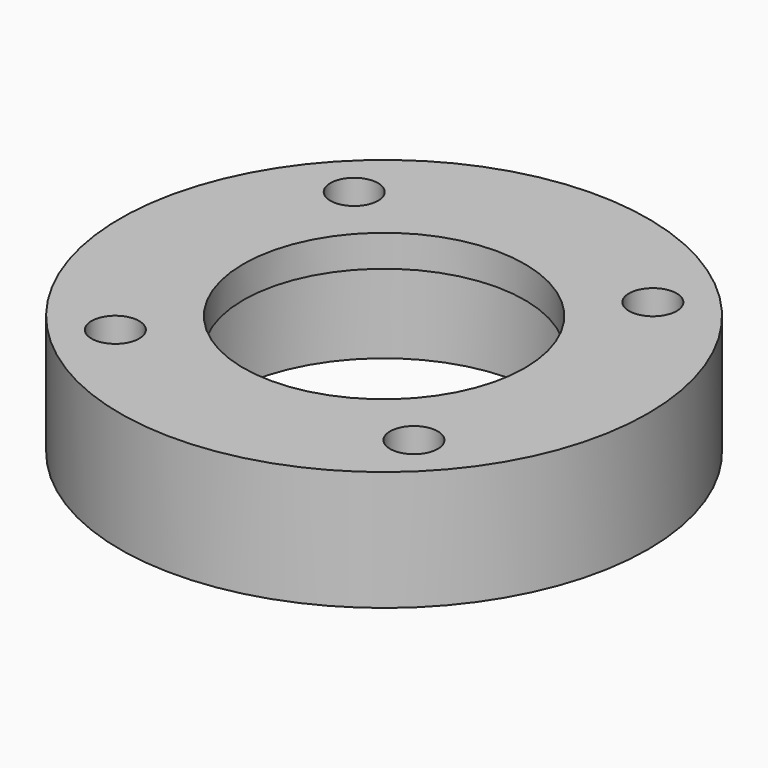
from build123d import *

# Parameters (mm, degrees)
F0_R            = 23.8125
F0_R_2          = 2.15265
F0_R_3          = 14.2875
F1_DEPTH        = 7.9375
F3_DEPTH        = 7.9375
F3_COPIES_COUNT = 4
F4_R            = 23.8125
F4_R_2          = 2.15265
F4_R_3          = 14.2875
F4_R_4          = 12.7
F5_DEPTH        = 2.8575


# Not quite as in the source:
# - a pattern or mirror of a feature is missing from the dataset's text; its kind, count and spacing are read off the source's solid


with BuildPart() as f1:
    # F0 (on Top) → F1 (new body)
    with BuildSketch(Plane.XY):
        Circle(F0_R)
        with Locations((-13.4703841816, -13.4703841816)):
            Circle(F0_R_2, mode=Mode.SUBTRACT)
        with Locations((13.4703841816, -13.4703841816)):
            Circle(F0_R_2, mode=Mode.SUBTRACT)
        with Locations((-13.4703841816, 13.4703841816)):
            Circle(F0_R_2, mode=Mode.SUBTRACT)
        Circle(F0_R_3, mode=Mode.SUBTRACT)
        with Locations((13.4703841816, 13.4703841816)):
            Circle(F0_R_2, mode=Mode.SUBTRACT)
    extrude(amount=F1_DEPTH)

    # F2 (on face) → F3 (cut, through all)
    with BuildSketch(Plane.XY.offset(7.9375)):
        with BuildLine():
            ThreePointArc((12.7805200237, -18.1826547271), (10.4181406182, -17.1262309344), (8.9569606825, -14.9903889737))
            ThreePointArc((8.9569606825, -14.9903889737), (0, -17.4625), (-8.9569606825, -14.9903889737))
            ThreePointArc((-8.9569606825, -14.9903889737), (-10.4181406182, -17.1262309344), (-12.7805200237, -18.1826547271))
            ThreePointArc((-12.7805200237, -18.1826547271), (0, -22.225), (12.7805200237, -18.1826547271))
        make_face()
    f3 = extrude(amount=-F3_DEPTH, mode=Mode.SUBTRACT)

    # F3_copies: F3 ×4 about axis
    f3_copies_axis = Axis((0, 0, 0), (0, 0, 1))
    for i in range(1, F3_COPIES_COUNT):
        add(f3.rotate(f3_copies_axis, i * 360 / F3_COPIES_COUNT), mode=Mode.SUBTRACT)

    # F4 (on face) → F5 (join)
    with BuildSketch(Plane.XY.offset(7.9375)):
        Circle(F4_R)
        with Locations((-13.4703841816, -13.4703841816)):
            Circle(F4_R_2, mode=Mode.SUBTRACT)
        with BuildLine():
            ThreePointArc((-8.9569606825, -14.9903889737), (0, -17.4625), (8.9569606825, -14.9903889737))
            ThreePointArc((8.9569606825, -14.9903889737), (10.4181406182, -17.1262309344), (12.7805200237, -18.1826547271))
            ThreePointArc((12.7805200237, -18.1826547271), (0, -22.225), (-12.7805200237, -18.1826547271))
            ThreePointArc((-12.7805200237, -18.1826547271), (-10.4181406182, -17.1262309344), (-8.9569606825, -14.9903889737))
        make_face(mode=Mode.SUBTRACT)
        with Locations((13.4703841816, -13.4703841816)):
            Circle(F4_R_2, mode=Mode.SUBTRACT)
        with BuildLine():
            ThreePointArc((-14.9903889737, 8.9569606825), (-17.4625, 0), (-14.9903889737, -8.9569606825))
            ThreePointArc((-14.9903889737, -8.9569606825), (-17.1262309344, -10.4181406182), (-18.1826547271, -12.7805200237))
            ThreePointArc((-18.1826547271, -12.7805200237), (-22.225, 0), (-18.1826547271, 12.7805200237))
            ThreePointArc((-18.1826547271, 12.7805200237), (-17.1262309344, 10.4181406182), (-14.9903889737, 8.9569606825))
        make_face(mode=Mode.SUBTRACT)
        with Locations((-13.4703841816, 13.4703841816)):
            Circle(F4_R_2, mode=Mode.SUBTRACT)
        Circle(F4_R_3, mode=Mode.SUBTRACT)
        with BuildLine():
            ThreePointArc((14.9903889737, -8.9569606825), (17.4625, 0), (14.9903889737, 8.9569606825))
            ThreePointArc((14.9903889737, 8.9569606825), (17.1262309344, 10.4181406182), (18.1826547271, 12.7805200237))
            ThreePointArc((18.1826547271, 12.7805200237), (22.225, 0), (18.1826547271, -12.7805200237))
            ThreePointArc((18.1826547271, -12.7805200237), (17.1262309344, -10.4181406182), (14.9903889737, -8.9569606825))
        make_face(mode=Mode.SUBTRACT)
        with BuildLine():
            ThreePointArc((8.9569606825, 14.9903889737), (0, 17.4625), (-8.9569606825, 14.9903889737))
            ThreePointArc((-8.9569606825, 14.9903889737), (-10.4181406182, 17.1262309344), (-12.7805200237, 18.1826547271))
            ThreePointArc((-12.7805200237, 18.1826547271), (0, 22.225), (12.7805200237, 18.1826547271))
            ThreePointArc((12.7805200237, 18.1826547271), (10.4181406182, 17.1262309344), (8.9569606825, 14.9903889737))
        make_face(mode=Mode.SUBTRACT)
        with Locations((13.4703841816, 13.4703841816)):
            Circle(F4_R_2, mode=Mode.SUBTRACT)
        with BuildLine():
            ThreePointArc((12.7805200237, -18.1826547271), (10.4181406182, -17.1262309344), (8.9569606825, -14.9903889737))
            ThreePointArc((8.9569606825, -14.9903889737), (0, -17.4625), (-8.9569606825, -14.9903889737))
            ThreePointArc((-8.9569606825, -14.9903889737), (-10.4181406182, -17.1262309344), (-12.7805200237, -18.1826547271))
            ThreePointArc((-12.7805200237, -18.1826547271), (0, -22.225), (12.7805200237, -18.1826547271))
        make_face()
        with BuildLine():
            ThreePointArc((-18.1826547271, -12.7805200237), (-17.1262309344, -10.4181406182), (-14.9903889737, -8.9569606825))
            ThreePointArc((-14.9903889737, -8.9569606825), (-17.4625, 0), (-14.9903889737, 8.9569606825))
            ThreePointArc((-14.9903889737, 8.9569606825), (-17.1262309344, 10.4181406182), (-18.1826547271, 12.7805200237))
            ThreePointArc((-18.1826547271, 12.7805200237), (-22.225, 0), (-18.1826547271, -12.7805200237))
        make_face()
        Circle(F4_R_3)
        Circle(F4_R_4, mode=Mode.SUBTRACT)
        with BuildLine():
            ThreePointArc((18.1826547271, 12.7805200237), (17.1262309344, 10.4181406182), (14.9903889737, 8.9569606825))
            ThreePointArc((14.9903889737, 8.9569606825), (17.4625, 0), (14.9903889737, -8.9569606825))
            ThreePointArc((14.9903889737, -8.9569606825), (17.1262309344, -10.4181406182), (18.1826547271, -12.7805200237))
            ThreePointArc((18.1826547271, -12.7805200237), (22.225, 0), (18.1826547271, 12.7805200237))
        make_face()
        with BuildLine():
            ThreePointArc((-12.7805200237, 18.1826547271), (-10.4181406182, 17.1262309344), (-8.9569606825, 14.9903889737))
            ThreePointArc((-8.9569606825, 14.9903889737), (0, 17.4625), (8.9569606825, 14.9903889737))
            ThreePointArc((8.9569606825, 14.9903889737), (10.4181406182, 17.1262309344), (12.7805200237, 18.1826547271))
            ThreePointArc((12.7805200237, 18.1826547271), (0, 22.225), (-12.7805200237, 18.1826547271))
        make_face()
    extrude(amount=F5_DEPTH)


solid = f1.part
